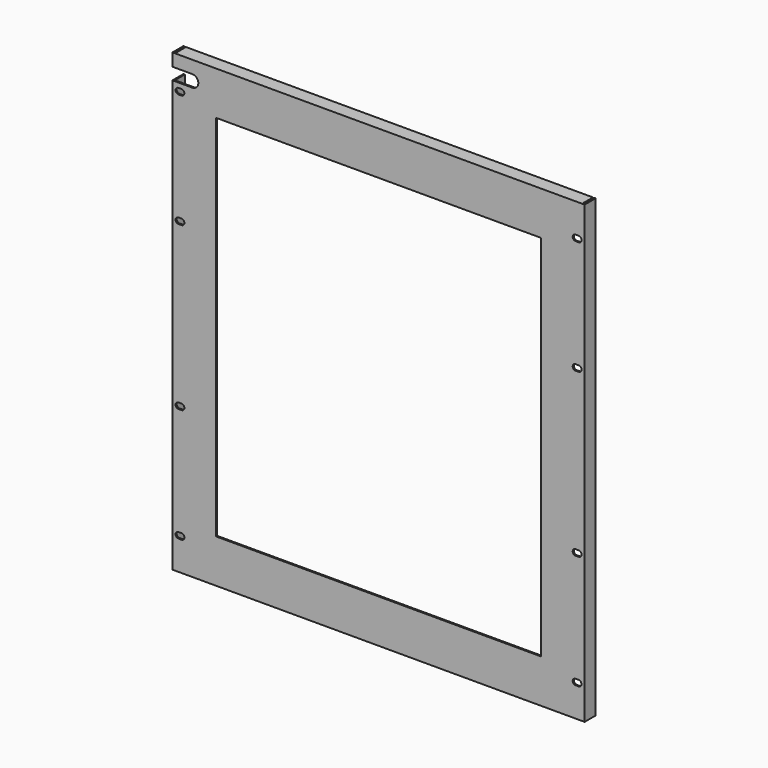
from build123d import *

# Parameters (mm, degrees)
F0_W              = 482.6
F0_H              = 533.2
F1_DEPTH          = 1.6
F2_W              = 16
F2_H              = 533.2
F3_DEPTH          = 1.6
F4_W              = 16
F4_H              = 533.2
F5_DEPTH          = 1.6
F6_W              = 476.6
F6_H              = 16
F7_DEPTH          = 1.6
F8_W              = 476.6
F8_H              = 16
F9_DEPTH          = 1.6
F10_W             = 381
F10_H             = 431.5
F11_DEPTH         = 1.6
F12_W             = 3.5
F12_H             = 6.8
F13_DEPTH         = 1.6
F13_COPIES3_COUNT = 2
F13_COPIES3_PITCH = 652.537999
F13_COPIES4_COUNT = 2
F13_COPIES4_PITCH = 566.888933
F14_W             = 3.5
F14_H             = 6.8
F15_DEPTH         = 1.6
F16_W             = 23.3
F16_H             = 14
F17_DEPTH         = 16


# Not quite as in the source:
# - a pattern or mirror of a feature is missing from the dataset's text; its kind, count and spacing are read off the source's solid


with BuildPart() as f1:
    # F0 (on Front) → F1 (new body)
    with BuildSketch(Plane.XZ):
        Rectangle(F0_W, F0_H)
    extrude(amount=-F1_DEPTH)

    # F2 (on face) → F3 (join)
    with BuildSketch(Plane(origin=(-241.3, 0, 0), x_dir=(0, -1, 0), z_dir=(-1, 0, 0))):
        with Locations((-8, 0)):
            Rectangle(F2_W, F2_H)
    extrude(amount=-F3_DEPTH)

    # F4 (on face) → F5 (join)
    with BuildSketch(Plane.YZ.offset(241.3)):
        with Locations((8, 0)):
            Rectangle(F4_W, F4_H)
    extrude(amount=-F5_DEPTH)

    # F6 (on face) → F7 (join)
    with BuildSketch(Plane.XY.offset(266.6)):
        with Locations((0, 8)):
            Rectangle(F6_W, F6_H)
    extrude(amount=-F7_DEPTH)

    # F8 (on face) → F9 (join)
    with BuildSketch(Plane(origin=(0, 0, -266.6), x_dir=(1, 0, 0), z_dir=(0, 0, -1))):
        with Locations((0, -8)):
            Rectangle(F8_W, F8_H)
    extrude(amount=-F9_DEPTH)

    # F10 (on face) → F11 (cut)
    with BuildSketch(Plane.XZ):
        Rectangle(F10_W, F10_H)
    extrude(amount=-F11_DEPTH, mode=Mode.SUBTRACT)

    # F12 (on face) → F13 (cut)
    with BuildSketch(Plane.XZ):
        with Locations((-232.5, -228.9)):
            Rectangle(F12_W, F12_H)
        with BuildLine():
            Line((-230.75, -225.5), (-230.75, -232.3))
            ThreePointArc((-230.75, -232.3), (-227.35, -228.9), (-230.75, -225.5))
        make_face()
        with BuildLine():
            ThreePointArc((-234.25, -225.5), (-237.65, -228.9), (-234.25, -232.3))
            Line((-234.25, -232.3), (-234.25, -225.5))
        make_face()
    f13 = extrude(amount=-F13_DEPTH, mode=Mode.SUBTRACT)

    # F13_copies: F13 across plane
    add(f13.mirror(Plane.XY), mode=Mode.SUBTRACT)

    # F13_copies1: F13 across plane
    add(f13.mirror(Plane.XY.offset(-66.775)), mode=Mode.SUBTRACT)

    # F13_copies2: F13 across plane
    add(f13.mirror(Plane(origin=(0, 0, 0), x_dir=(0, 0, 1), z_dir=(1, 0, 0))), mode=Mode.SUBTRACT)

    # F13_copies3: F13 ×2
    with Locations(*[Vector(0.7126021792, 0, 0.701568339) * (i * F13_COPIES3_PITCH) for i in range(1, F13_COPIES3_COUNT)]):
        add(f13, mode=Mode.SUBTRACT)

    # F13_copies4: F13 ×2
    with Locations(*[Vector(0.8202664981, 0, 0.5719815312) * (i * F13_COPIES4_PITCH) for i in range(1, F13_COPIES4_COUNT)]):
        add(f13, mode=Mode.SUBTRACT)

    # F14 (on face) → F15 (cut)
    with BuildSketch(Plane.XZ):
        with Locations((-232.5, -95.35)):
            Rectangle(F14_W, F14_H)
        with BuildLine():
            Line((-230.75, -91.95), (-230.75, -98.75))
            ThreePointArc((-230.75, -98.75), (-227.35, -95.35), (-230.75, -91.95))
        make_face()
        with BuildLine():
            ThreePointArc((-234.25, -91.95), (-237.65, -95.35), (-234.25, -98.75))
            Line((-234.25, -98.75), (-234.25, -91.95))
        make_face()
    f15 = extrude(amount=-F15_DEPTH, mode=Mode.SUBTRACT)

    # F15_copies: F15 across plane
    add(f15.mirror(Plane(origin=(0, 0, 0), x_dir=(0, 0, 1), z_dir=(1, 0, 0))), mode=Mode.SUBTRACT)

    # F16 (on face) → F17 (cut)
    with BuildSketch(Plane.XZ):
        with Locations((-229.65, 244.8)):
            Rectangle(F16_W, F16_H)
        with BuildLine():
            Line((-218, 251.8), (-218, 237.8))
            ThreePointArc((-218, 237.8), (-211, 244.8), (-218, 251.8))
        make_face()
    extrude(amount=-F17_DEPTH, mode=Mode.SUBTRACT)


solid = f1.part
